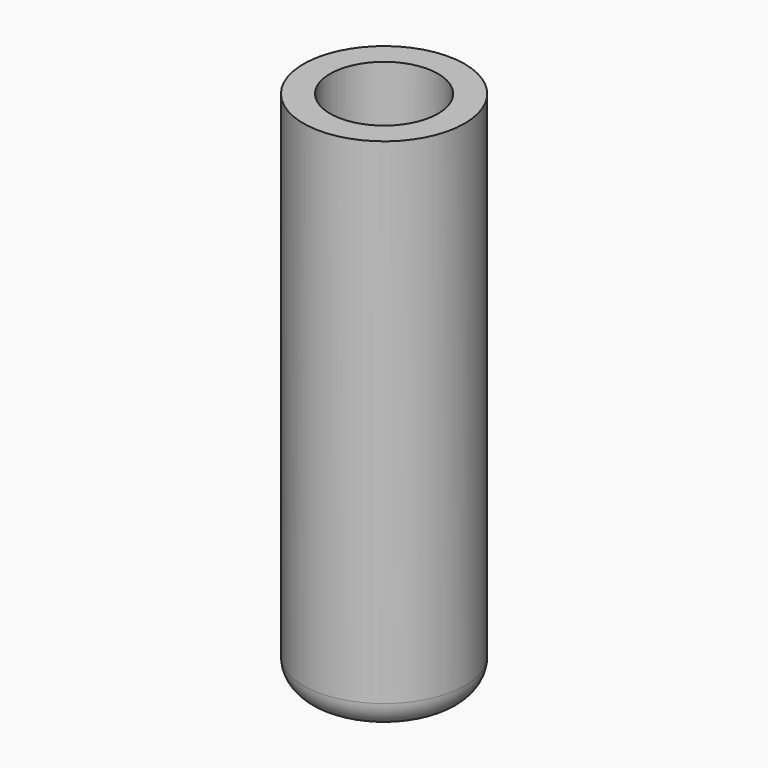
from build123d import *

# Parameters (mm, degrees)
F0_W = 7.6932697557
F0_H = 49.7964322567
F2_T = -2.54
F3_R = 2.53999


# Not quite as in the source:
# - a fillet or chamfer is up to 0.001 mm smaller than in the source, because OpenCascade refuses the exact size


with BuildPart() as f1:
    # F0 (on Front) → F1 (revolve)
    with BuildSketch(Plane.XZ):
        with Locations((3.8466348778, 4.3362062424)):
            Rectangle(F0_W, F0_H)
    revolve(axis=Axis((0, 0, 4.3362062424), (0, 0, -1)))

    # F2
    f2_openings = [f1.faces().sort_by_distance(p)[0] for p in [
        (0, 0, 29.234422),
        (0, 0, -20.56201),
    ]]
    offset(amount=F2_T, openings=f2_openings)

    # F3 (radius 2.54 in the source; OpenCascade refuses exactly that, so slightly less here)
    f3_edges = [f1.edges().sort_by_distance(p)[0] for p in [
        (-7.69327, 0, -20.56201),
    ]]
    fillet(f3_edges, radius=F3_R)


solid = f1.part
